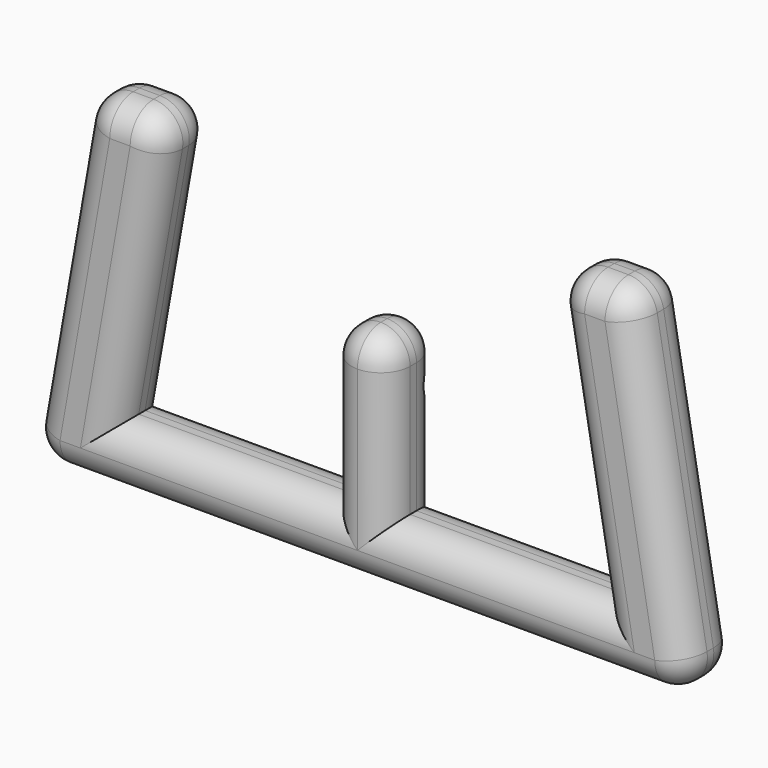
from build123d import *

# Parameters (mm, degrees)
F1_DEPTH = 25
F2_R     = 10.99999
F3_R     = 10
F4_DEPTH = 9.1


# Not quite as in the source:
# - a fillet or chamfer is up to 0.001 mm smaller than in the source, because OpenCascade refuses the exact size


with BuildPart() as f1:
    # F0 (on Front) → F1 (new body)
    with BuildSketch(Plane.XZ):
        Polygon((-104.7428149239, 128.0250078916), (-127.3170780206, 0), (122.4413091306, 0), (99.8670460339, 128.0250078916), (92.5590772594, 128.0250078916), (69.8670460339, 128.0250078916), (88.562115555, 22), (8.562115555, 22), (8.562115555, 82), (-13.437884445, 82), (-13.437884445, 22), (-93.437884445, 22), (-74.7428149239, 128.0250078916), (-93.565618156, 128.0250078916), align=None)
    extrude(amount=F1_DEPTH)

    # F2 (radius 11 in the source; OpenCascade refuses exactly that, so slightly less here)
    f2_edges = [f1.edges().sort_by_distance(p)[0] for p in [
        (-89.742815, -25, 128.025008),
        (-116.029946, -25, 64.012504),
        (-2.437884, -25, 0),
        (111.154178, -25, 64.012504),
        (84.867046, -25, 128.025008),
        (79.214581, -25, 75.012504),
        (48.562116, -25, 22),
        (8.562116, -25, 52),
        (-2.437884, -25, 82),
        (-13.437884, -25, 52),
        (-53.437884, -25, 22),
        (-84.09035, -25, 75.012504),
        (-89.742815, 0, 128.025008),
        (-116.029946, 0, 64.012504),
        (-2.437884, 0, 0),
        (111.154178, 0, 64.012504),
        (84.867046, 0, 128.025008),
        (79.214581, 0, 75.012504),
        (48.562116, 0, 22),
        (8.562116, 0, 52),
        (-2.437884, 0, 82),
        (-13.437884, 0, 52),
        (-53.437884, 0, 22),
        (-84.09035, 0, 75.012504),
        (-74.742815, -12.5, 128.025008),
        (-104.742815, -12.5, 128.025008),
        (8.562116, -12.5, 82),
        (-13.437884, -12.5, 82),
        (99.867046, -12.5, 128.025008),
        (69.867046, -12.5, 128.025008),
        (122.441309, -12.5, 0),
        (-127.317078, -12.5, 0),
    ]]
    fillet(f2_edges, radius=F2_R)

    # F3 (on Front) → F4 (cut)
    with BuildSketch(Plane.XZ):
        with Locations((-2.4443906732, 60.8239136636)):
            Circle(F3_R)
    extrude(amount=F4_DEPTH, mode=Mode.SUBTRACT)


solid = f1.part
